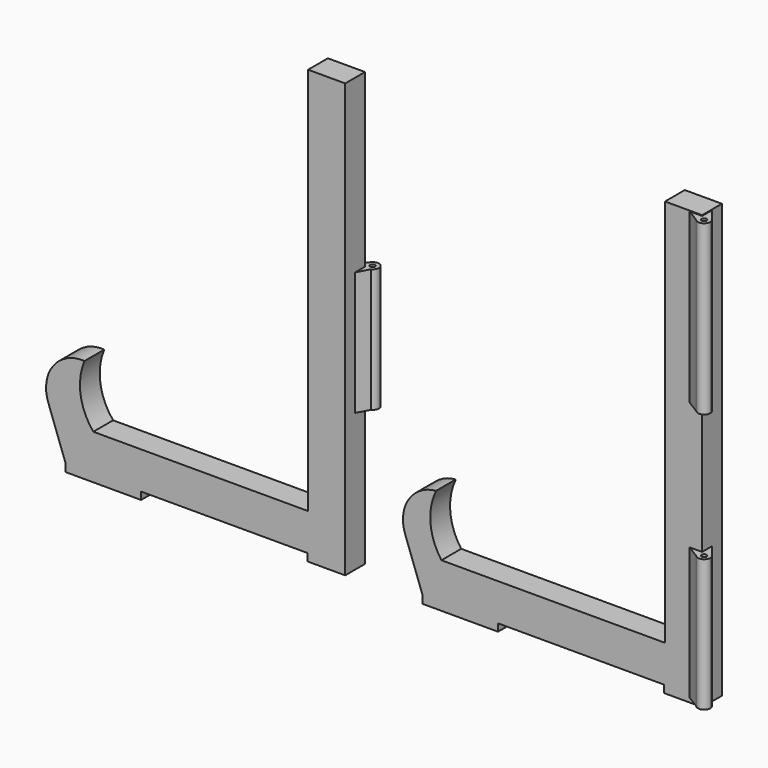
from build123d import *

# Parameters (mm, degrees)
F0_W          = 15.321185604
F0_H          = 3
F0_W_2        = 30.4560337395
F1_DEPTH      = 5
F2_R          = 1
F3_DEPTH      = 20
F3_DEPTH_BACK = 30
F4_START      = -20.5
F4_DEPTH      = 53.5
F5_START      = 31
F5_DEPTH      = 68


# Not quite as in the source:
# - a feature names something its author has since deleted; it is built from what else it names


with BuildPart() as f1:
    # F0 (on Front) → F1 (new body, symmetric)
    with BuildSketch(Plane.XZ):
        with BuildLine():
            Line((-142.8835457128, 99.2541786495), (-157.8835457128, 99.2541786495))
            Line((-157.8835457128, 99.2541786495), (-157.8835457128, -57.7458213505))
            Line((-157.8835457128, -57.7458213505), (-244.6652154244, -57.7458213505))
            ThreePointArc((-244.6652154244, -57.7458213505), (-249.819751502, -46.2428496856), (-248.2298080079, -33.7384632959))
            ThreePointArc((-248.2298080079, -33.7384632959), (-260.8309353496, -39.5226598893), (-262.8835457128, -53.2351407447))
            Line((-262.8835457128, -53.2351407447), (-255.8200499165, -72.7458213505))
            Line((-255.8200499165, -72.7458213505), (-225.3640161769, -72.7458213505))
            Line((-225.3640161769, -72.7458213505), (-158.2047313168, -72.7458213505))
            Line((-158.2047313168, -72.7458213505), (-142.8835457128, -72.7458213505))
            Line((-142.8835457128, -72.7458213505), (-142.8835457128, 99.2541786495))
        make_face()
        with Locations((-150.5441385148, -74.2458213505)):
            Rectangle(F0_W, F0_H)
        with Locations((-240.5920330467, -74.2458213505)):
            Rectangle(F0_W_2, F0_H)
    extrude(amount=F1_DEPTH, both=True)


with BuildPart() as f1b:
    # F0 (on Front) → F1, piece 2 (new body, symmetric)
    with BuildSketch(Plane.XZ):
        with BuildLine():
            Line((1.3299961225, 99.2861494968), (-13.6700038775, 99.2861494968))
            Line((-13.6700038775, 99.2861494968), (-13.6700038775, -57.7138505032))
            Line((-13.6700038775, -57.7138505032), (-104.0030368801, -57.7138505032))
            ThreePointArc((-104.0030368801, -57.7138505032), (-108.4245444734, -46.0201943036), (-106.1661484389, -33.7242204885))
            ThreePointArc((-106.1661484389, -33.7242204885), (-117.2315141427, -40.373870816), (-118.6700038775, -53.2031698974))
            Line((-118.6700038775, -53.2031698974), (-111.6065080813, -72.7138505032))
            Line((-111.6065080813, -72.7138505032), (-81.1504743417, -72.7138505032))
            Line((-81.1504743417, -72.7138505032), (-13.9911894815, -72.7138505032))
            Line((-13.9911894815, -72.7138505032), (1.3299961225, -72.7138505032))
            Line((1.3299961225, -72.7138505032), (1.3299961225, -2.6822620718))
            Line((1.3299961225, -2.6822620718), (1.3299961225, 31.9242632935))
            Line((1.3299961225, 31.9242632935), (1.3299961225, 99.2861494968))
        make_face()
        with Locations((-96.3784912115, -74.2138505032)):
            Rectangle(F0_W_2, F0_H)
        with Locations((-6.3305966795, -74.2138505032)):
            Rectangle(F0_W, F0_H)
    extrude(amount=F1_DEPTH, both=True)

    # F2 (on Top) → F4 (join)
    with BuildSketch(Plane.XY.offset(F4_START)):
        with BuildLine():
            ThreePointArc((1.5607074298, -8.2591902465), (4.3176765393, -8.9350586961), (5.9292119056, -6.598259476))
            ThreePointArc((5.9292119056, -6.598259476), (5.6531681475, -5.4563231231), (4.8859969983, -4.5665662921))
            ThreePointArc((4.8859969983, -4.5665662921), (1.5941978234, -4.9004010255), (1.5165762661, -8.2081740423))
            ThreePointArc((1.5165762661, -8.2081740423), (1.5384697746, -8.2338309951), (1.5607074298, -8.2591902465))
        make_face()
        with Locations((3.4292119056, -6.598259476)):
            Circle(F2_R, mode=Mode.SUBTRACT)
        with BuildLine():
            ThreePointArc((1.5165762661, -8.2081740423), (1.5941978234, -4.9004010255), (4.8859969983, -4.5665662921))
            Line((4.8859969983, -4.5665662921), (1.3131950982, 0))
            Line((1.3131950982, 0), (-3.6700038775, -5.0244089216))
            Line((-3.6700038775, -5.0244089216), (1.5165762661, -8.2081740423))
        make_face()
        with BuildLine():
            Line((-3.6700038775, -5.0244089216), (1.5607074298, -8.2591902465))
            ThreePointArc((1.5607074298, -8.2591902465), (1.5384697746, -8.2338309951), (1.5165762661, -8.2081740423))
            Line((1.5165762661, -8.2081740423), (-3.6700038775, -5.0244089216))
        make_face()
    extrude(amount=-F4_DEPTH)


with BuildPart() as f3:
    # F2 (on Top) → F3 (new body, two sides)
    with BuildSketch(Plane.XY) as f3_sk:
        with BuildLine():
            ThreePointArc((-140.3050830614, 4.7814064547), (-139.2797249014, 5.7036192761), (-138.8993577326, 7.0291971353))
            ThreePointArc((-138.8993577326, 7.0291971353), (-140.7523801028, 9.4440304518), (-143.5644936898, 8.2790716438))
            ThreePointArc((-143.5644936898, 8.2790716438), (-143.228319574, 5.3248208322), (-140.3050830614, 4.7814064547))
        make_face()
        with Locations((-141.3993577326, 7.0291971353)):
            Circle(F2_R, mode=Mode.SUBTRACT)
        with BuildLine():
            ThreePointArc((-140.3050830614, 4.7814064547), (-143.228319574, 5.3248208322), (-143.5644936898, 8.2790716438))
            Line((-143.5644936898, 8.2790716438), (-147.8835457128, 4.9874218958))
            Line((-147.8835457128, 4.9874218958), (-142.8794413805, 0))
            Line((-142.8794413805, 0), (-140.3050830614, 4.7814064547))
        make_face()
    extrude(amount=-F3_DEPTH)
    extrude(f3_sk.sketch, amount=F3_DEPTH_BACK)


with BuildPart() as f5:
    # F2 (on Top) → F5 (new body)
    with BuildSketch(Plane.XY.offset(F5_START)):
        with BuildLine():
            ThreePointArc((1.5607074298, -8.2591902465), (4.3176765393, -8.9350586961), (5.9292119056, -6.598259476))
            ThreePointArc((5.9292119056, -6.598259476), (5.6531681475, -5.4563231231), (4.8859969983, -4.5665662921))
            ThreePointArc((4.8859969983, -4.5665662921), (1.5941978234, -4.9004010255), (1.5165762661, -8.2081740423))
            ThreePointArc((1.5165762661, -8.2081740423), (1.5384697746, -8.2338309951), (1.5607074298, -8.2591902465))
        make_face()
        with Locations((3.4292119056, -6.598259476)):
            Circle(F2_R, mode=Mode.SUBTRACT)
        with BuildLine():
            ThreePointArc((1.5165762661, -8.2081740423), (1.5941978234, -4.9004010255), (4.8859969983, -4.5665662921))
            Line((4.8859969983, -4.5665662921), (1.3131950982, 0))
            Line((1.3131950982, 0), (-3.6700038775, -5.0244089216))
            Line((-3.6700038775, -5.0244089216), (1.5165762661, -8.2081740423))
        make_face()
        with BuildLine():
            Line((-3.6700038775, -5.0244089216), (1.5607074298, -8.2591902465))
            ThreePointArc((1.5607074298, -8.2591902465), (1.5384697746, -8.2338309951), (1.5165762661, -8.2081740423))
            Line((1.5165762661, -8.2081740423), (-3.6700038775, -5.0244089216))
        make_face()
    extrude(amount=F5_DEPTH)


solid = Compound([f1.part, f1b.part, f3.part, f5.part])
